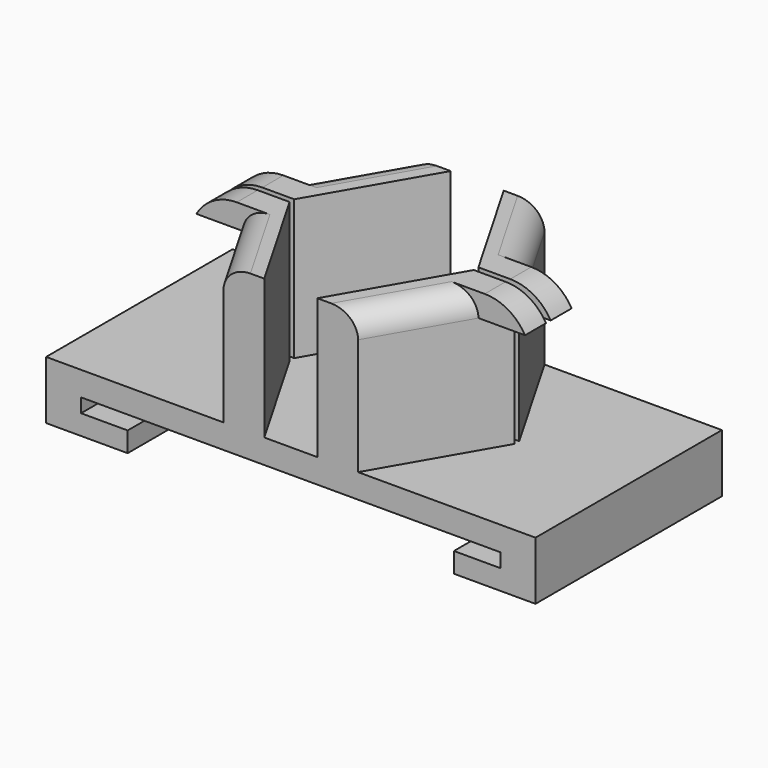
from build123d import *

# Parameters (mm, degrees)
F1_DEPTH    = 10
F3_DEPTH    = 6
F6_DEPTH    = 1
F7_DEPTH    = 1
F8_T1_DEPTH = 11.1602540378
F9_R        = 1
F10_W       = 3.6315133076
F10_H       = 0.25
F11_DEPTH   = 6
F12_W       = 3.6315133076
F12_H       = 0.25
F13_DEPTH   = 6


# Not quite as in the source:
# - a fillet or chamfer that OpenCascade refuses, or shapes differently, is made with other operations: its cross-section is extruded or revolved along the edge and cut away or added


with BuildPart() as f1:
    # F0 (on Front) → F1 (new body)
    with BuildSketch(Plane.XZ):
        Polygon((7, -1.25), (10.5, -1.25), (10.5, 1.25), (-10.5, 1.25), (-10.5, -1.25), (-7, -1.25), (-7, -0.3903658071), (-9, -0.3903658071), (-9, 0.2096341929), (9, 0.2096341929), (9, -0.3903658071), (7, -0.3903658071), align=None)
    extrude(amount=F1_DEPTH)

    # F2 (on face) → F3 (join)
    with BuildSketch(Plane.XY.offset(1.25)):
        Polygon((-1.137, -10), (-4.0235, -5), (-5.7735, -5), (-2.887, -10), align=None)
        Polygon((-4.0235, -5), (-1.137, 0), (-2.887, 0), (-5.7735, -5), align=None)
        Polygon((2.887, 0), (1.137, 0), (4.0235, -5), (5.7735, -5), align=None)
        Polygon((5.7735, -5), (4.0235, -5), (1.137, -10), (2.887, -10), align=None)
    extrude(amount=F3_DEPTH)

    # F4 (on face) → F6 (join)
    with BuildSketch(Plane.XY.offset(7.25)):
        Polygon((-5.7735, -5), (-5.051875, -3.75), (-7.051875, -3.75), (-7.051875, -6.25), (-5.051875, -6.25), align=None)
    extrude(amount=-F6_DEPTH)

    # F5 (on face) → F7 (join)
    with BuildSketch(Plane.XY.offset(7.25)):
        Polygon((7.051875, -3.75), (5.051875, -3.75), (5.7735, -5), (5.051875, -6.25), (7.051875, -6.25), align=None)
    extrude(amount=-F7_DEPTH)

    # F8: fillet of radius 2 on 2 edges, made by hand

    # F8_s2 → F8_t1 (cut)
    with BuildSketch(Plane.XZ.offset(-0.5801270189)):
        with BuildLine():
            ThreePointArc((-5.3198241924, 7.25), (-6.3198241924, 6.9820508076), (-7.051875, 6.25))
            Line((-7.051875, 6.25), (-7.051875, 7.25))
            Line((-7.051875, 7.25), (-5.3198241924, 7.25))
        make_face()
        with BuildLine():
            ThreePointArc((5.3198241924, 7.25), (6.3198241924, 6.9820508076), (7.051875, 6.25))
            Line((7.051875, 6.25), (7.051875, 7.25))
            Line((7.051875, 7.25), (5.3198241924, 7.25))
        make_face()
    extrude(amount=F8_T1_DEPTH, mode=Mode.SUBTRACT)

    # F9
    f9_edges = [f1.edges().sort_by_distance(p)[0] for p in [
        (-3.969438, -8.125, 7.25),
        (-3.969438, -1.875, 7.25),
        (3.969437, -8.125, 7.25),
        (3.969437, -1.875, 7.25),
    ]]
    fillet(f9_edges, radius=F9_R)

    # F10 (on face) → F11 (cut)
    with BuildSketch(Plane.XY.offset(7.25)):
        Polygon((-4.0235, -5), (-3.9513375, -4.875), (-5.3198241924, -4.875), (-5.3198241924, -5.125), (-3.9513375, -5.125), align=None)
        with Locations((-7.1355808462, -5)):
            Rectangle(F10_W, F10_H)
    extrude(amount=-F11_DEPTH, mode=Mode.SUBTRACT)

    # F12 (on face) → F13 (cut)
    with BuildSketch(Plane.XY.offset(7.25)):
        with Locations((7.1355808462, -5)):
            Rectangle(F12_W, F12_H)
        Polygon((5.3198241924, -4.875), (3.9513375, -4.875), (4.0235, -5), (3.9513375, -5.125), (5.3198241924, -5.125), align=None)
    extrude(amount=-F13_DEPTH, mode=Mode.SUBTRACT)


solid = f1.part
